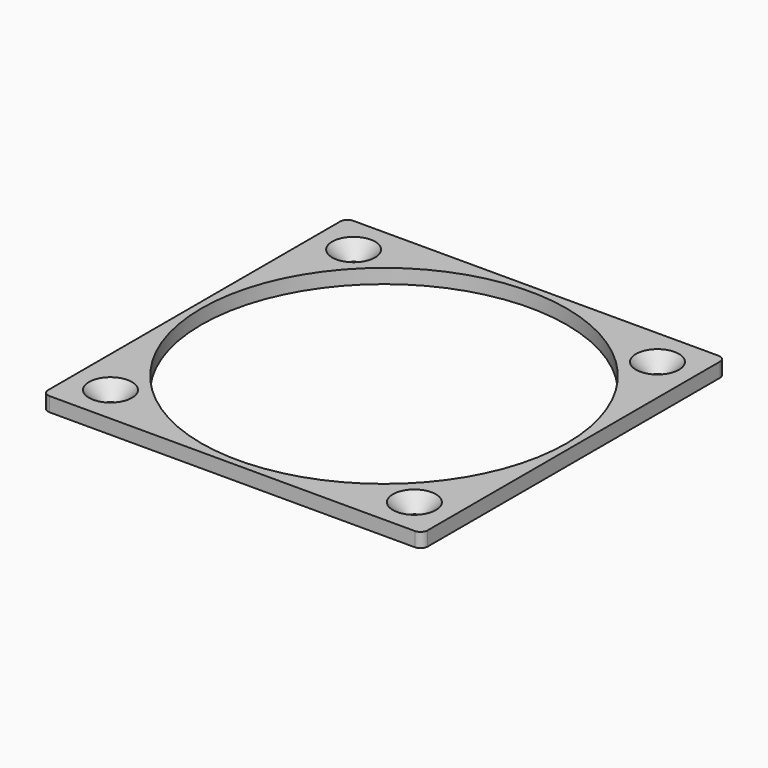
from build123d import *

# Parameters (mm, degrees)
F0_W     = 53
F0_H     = 53
F0_R     = 1
F0_R_2   = 25.5
F1_DEPTH = 2
F2_SIZE  = 1.99999
F3_R     = 1


# Not quite as in the source:
# - a fillet or chamfer is up to 0.001 mm smaller than in the source, because OpenCascade refuses the exact size


with BuildPart() as f1:
    # F0 (on Top) → F1 (new body)
    with BuildSketch(Plane.XY):
        Rectangle(F0_W, F0_H)
        with Locations((-21.2132034356, -21.2132034356)):
            Circle(F0_R, mode=Mode.SUBTRACT)
        with Locations((21.2132034356, -21.2132034356)):
            Circle(F0_R, mode=Mode.SUBTRACT)
        with Locations((-21.2132034356, 21.2132034356)):
            Circle(F0_R, mode=Mode.SUBTRACT)
        Circle(F0_R_2, mode=Mode.SUBTRACT)
        with Locations((21.2132034356, 21.2132034356)):
            Circle(F0_R, mode=Mode.SUBTRACT)
    extrude(amount=F1_DEPTH)

    # F2 (size 2 in the source; OpenCascade refuses exactly that, so slightly less here)
    f2_edges = [f1.edges().sort_by_distance(p)[0] for p in [
        (-22.213203, 21.213203, 2),
        (20.213203, 21.213203, 2),
        (20.213203, -21.213203, 2),
        (-22.213203, -21.213203, 2),
    ]]
    chamfer(f2_edges, length=F2_SIZE)

    # F3
    f3_edges = [f1.edges().sort_by_distance(p)[0] for p in [
        (26.5, -26.5, 1),
        (26.5, 26.5, 1),
        (-26.5, -26.5, 1),
        (-26.5, 26.5, 1),
    ]]
    fillet(f3_edges, radius=F3_R)


solid = f1.part
